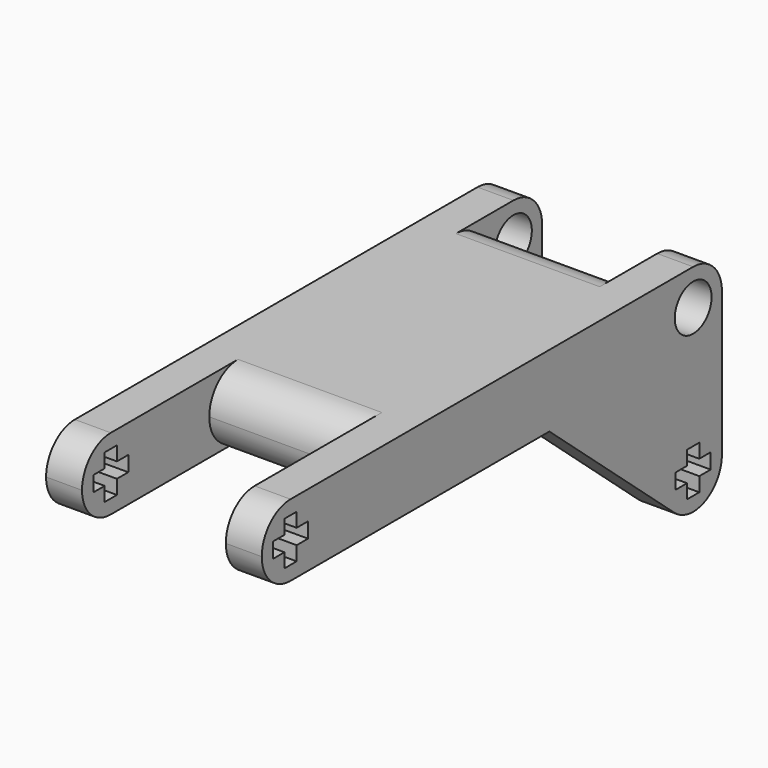
from build123d import *

# Parameters (mm, degrees)
F1_DEPTH = 7.9375
F2_R     = 3.96874
F3_W     = 3.96875
F3_H     = 23.8125
F4_DEPTH = 15.875
F5_W     = 1.56845
F5_H     = 1.6891
F5_W_2   = 1.6891
F5_H_2   = 1.56845
F5_R     = 2.54
F6_DEPTH = 23.8125


# Not quite as in the source:
# - a fillet or chamfer is up to 0.001 mm smaller than in the source, because OpenCascade refuses the exact size


with BuildPart() as f1:
    # F0 (on Top) → F1 (new body)
    with BuildSketch(Plane.XY):
        Polygon((0, 63.5), (0, 0), (3.96875, 0), (3.96875, 17.5562514), (19.84375, 17.5562514), (19.84375, 0), (23.8125, 0), (23.8125, 63.5), (19.84375, 63.5), (19.84375, 55.5625), (3.96875, 55.5625), (3.96875, 63.5), align=None)
    extrude(amount=F1_DEPTH)

    # F2 (radius 3.96875 in the source; OpenCascade refuses exactly that, so slightly less here)
    f2_edges = [f1.edges().sort_by_distance(p)[0] for p in [
        (11.90625, 55.5625, 7.9375),
        (11.90625, 55.5625, 0),
        (1.984375, 63.5, 7.9375),
        (21.828125, 63.5, 7.9375),
        (1.984375, 0, 7.9375),
        (1.984375, 0, 0),
        (21.828125, 0, 7.9375),
        (21.828125, 0, 0),
        (11.90625, 17.556251, 7.9375),
        (11.90625, 17.556251, 0),
    ]]
    fillet(f2_edges, radius=F2_R)

    # F3 (on face) → F4 (join)
    with BuildSketch(Plane(origin=(0, 0, 0), x_dir=(1, 0, 0), z_dir=(0, 0, -1))):
        with Locations((21.828125, -51.59375)):
            Rectangle(F3_W, F3_H)
        with Locations((1.984375, -51.59375)):
            Rectangle(F3_W, F3_H)
    extrude(amount=F4_DEPTH)

    # F5 (on face) → F6 (cut, through all)
    with BuildSketch(Plane(origin=(0, 0, 0), x_dir=(0, -1, 0), z_dir=(-1, 0, 0))):
        with Locations((-5.597525, 3.96875)):
            Rectangle(F5_W, F5_H)
        with Locations((-3.96875, 3.96875)):
            Rectangle(F5_W_2, F5_H)
        with Locations((-3.96875, 2.339975)):
            Rectangle(F5_W_2, F5_H_2)
        with Locations((-2.339975, 3.96875)):
            Rectangle(F5_W, F5_H)
        with Locations((-3.96875, 5.597525)):
            Rectangle(F5_W_2, F5_H_2)
        with BuildLine():
            Line((-63.5, -15.875), (-59.53125, -15.875))
            ThreePointArc((-59.53125, -15.875), (-62.3375800378, -14.7125800378), (-63.5, -11.90625))
            Line((-63.5, -11.90625), (-63.5, -15.875))
        make_face()
        with BuildLine():
            Line((-59.53125, -15.875), (-39.6875, -15.875))
            Line((-39.6875, -15.875), (-39.6875, 0))
            Line((-39.6875, 0), (-56.935957382, -14.9088210299))
            ThreePointArc((-56.935957382, -14.9088210299), (-58.146597916, -15.6256202651), (-59.53125, -15.875))
        make_face()
        with Locations((-57.902475, -11.90625)):
            Rectangle(F5_W, F5_H)
        with Locations((-59.53125, -11.90625)):
            Rectangle(F5_W_2, F5_H)
        with Locations((-59.53125, -10.277475)):
            Rectangle(F5_W_2, F5_H_2)
        with Locations((-61.160025, -11.90625)):
            Rectangle(F5_W, F5_H)
        with Locations((-59.53125, -13.535025)):
            Rectangle(F5_W_2, F5_H_2)
        with Locations((-59.53125, 3.96875)):
            Circle(F5_R)
    extrude(amount=-F6_DEPTH, mode=Mode.SUBTRACT)


solid = f1.part
